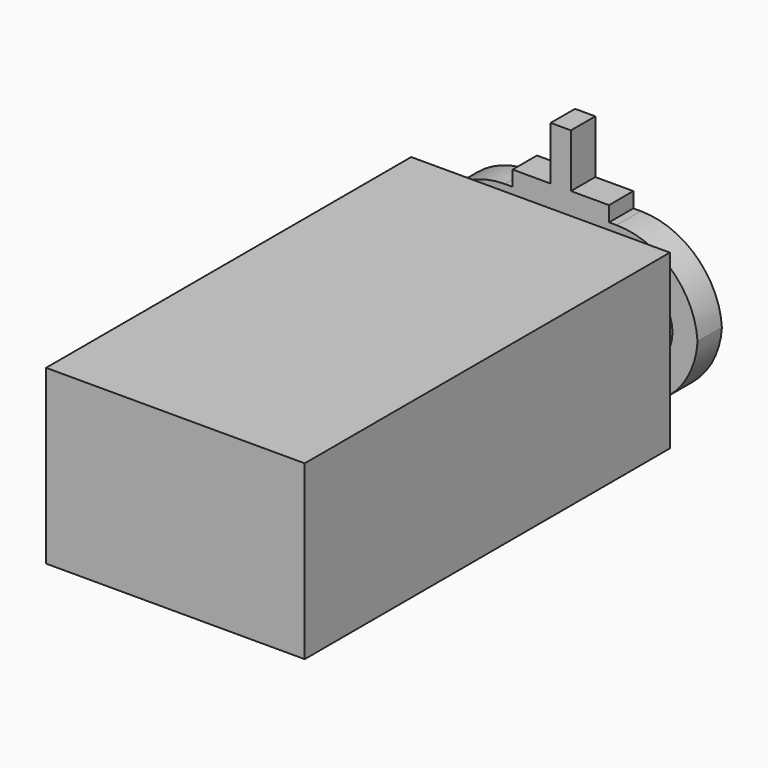
from build123d import *

# Parameters (mm, degrees)
F0_W         = 25.5
F0_H         = 45
F1_DEPTH     = 8.5
F2_R         = 2.5
F2_R_2       = 4
F3_DEPTH     = 2.5
F5_DEPTH     = 3
F6_T4_DEPTH  = 43
F6_T9_DEPTH  = 43
F6_T14_DEPTH = 43
F6_T19_DEPTH = 43


# Not quite as in the source:
# - a fillet or chamfer that OpenCascade refuses, or shapes differently, is made with other operations: its cross-section is extruded or revolved along the edge and cut away or added


with BuildPart() as f1:
    # F0 (on Top) → F1 (new body, symmetric)
    with BuildSketch(Plane.XY):
        with Locations((0, -1.3867942244)):
            Rectangle(F0_W, F0_H)
    extrude(amount=F1_DEPTH, both=True)

    # F2 (on face) → F3 (join)
    with BuildSketch(Plane(origin=(0, 21.1132057756, 0), x_dir=(-1, 0, 0), z_dir=(0, 1, 0))):
        with Locations((6, 0)):
            Circle(F2_R)
        with Locations((-7, 0)):
            Circle(F2_R_2)
    extrude(amount=F3_DEPTH)

    # F4 (on face) → F5 (join)
    with BuildSketch(Plane(origin=(0, 23.6132057756, 0), x_dir=(-1, 0, 0), z_dir=(0, 1, 0))):
        Polygon((-4.75, 7.5), (-13.5, 7.5), (-13.5, -7.5), (13.5, -7.5), (13.5, 7.5), (4.75, 7.5), (4.75, 9), (1, 9), (1, 14.2706949264), (-1, 14.2706949264), (-1, 9), (-4.75, 9), align=None)
    extrude(amount=F5_DEPTH)

    # F6: fillet of radius 8 on 4 edges, made by hand


with BuildPart() as f6_tool2:
    # F6_s3 → F6_t4 (new body)
    with BuildSketch(Plane.XZ.offset(-3.6132057756)):
        with BuildLine():
            ThreePointArc((5.5, 7.5), (11.1568542495, 5.1568542495), (13.5, -0.5))
            Line((13.5, -0.5), (13.5, 7.5))
            Line((13.5, 7.5), (5.5, 7.5))
        make_face()
    extrude(amount=-F6_T4_DEPTH)

    split(bisect_by=Plane.XZ.offset(-21.1132057756), keep=Keep.BOTTOM)


with BuildPart() as f1_1:
    add(f1.part)

    # F6_t1: cut F6_tool2
    add(f6_tool2.part, mode=Mode.SUBTRACT)


with BuildPart() as f6_tool7:
    # F6_s8 → F6_t9 (new body)
    with BuildSketch(Plane.XZ.offset(-3.6132057756)):
        with BuildLine():
            ThreePointArc((-13.5, -0.5), (-11.1568542495, 5.1568542495), (-5.5, 7.5))
            Line((-5.5, 7.5), (-13.5, 7.5))
            Line((-13.5, 7.5), (-13.5, -0.5))
        make_face()
    extrude(amount=-F6_T9_DEPTH)

    split(bisect_by=Plane.XZ.offset(-21.1132057756), keep=Keep.BOTTOM)


with BuildPart() as f1_2:
    add(f1_1.part)

    # F6_t6: cut F6_tool7
    add(f6_tool7.part, mode=Mode.SUBTRACT)


with BuildPart() as f6_tool12:
    # F6_s13 → F6_t14 (new body)
    with BuildSketch(Plane.XZ.offset(-3.6132057756)):
        with BuildLine():
            ThreePointArc((-5.5, -7.5), (-11.1568542495, -5.1568542495), (-13.5, 0.5))
            Line((-13.5, 0.5), (-13.5, -7.5))
            Line((-13.5, -7.5), (-5.5, -7.5))
        make_face()
    extrude(amount=-F6_T14_DEPTH)

    split(bisect_by=Plane.XZ.offset(-21.1132057756), keep=Keep.BOTTOM)


with BuildPart() as f1_3:
    add(f1_2.part)

    # F6_t11: cut F6_tool12
    add(f6_tool12.part, mode=Mode.SUBTRACT)


with BuildPart() as f6_tool17:
    # F6_s18 → F6_t19 (new body)
    with BuildSketch(Plane.XZ.offset(-3.6132057756)):
        with BuildLine():
            ThreePointArc((13.5, 0.5), (11.1568542495, -5.1568542495), (5.5, -7.5))
            Line((5.5, -7.5), (13.5, -7.5))
            Line((13.5, -7.5), (13.5, 0.5))
        make_face()
    extrude(amount=-F6_T19_DEPTH)

    split(bisect_by=Plane.XZ.offset(-21.1132057756), keep=Keep.BOTTOM)


with BuildPart() as f1_4:
    add(f1_3.part)

    # F6_t16: cut F6_tool17
    add(f6_tool17.part, mode=Mode.SUBTRACT)


solid = f1_4.part
